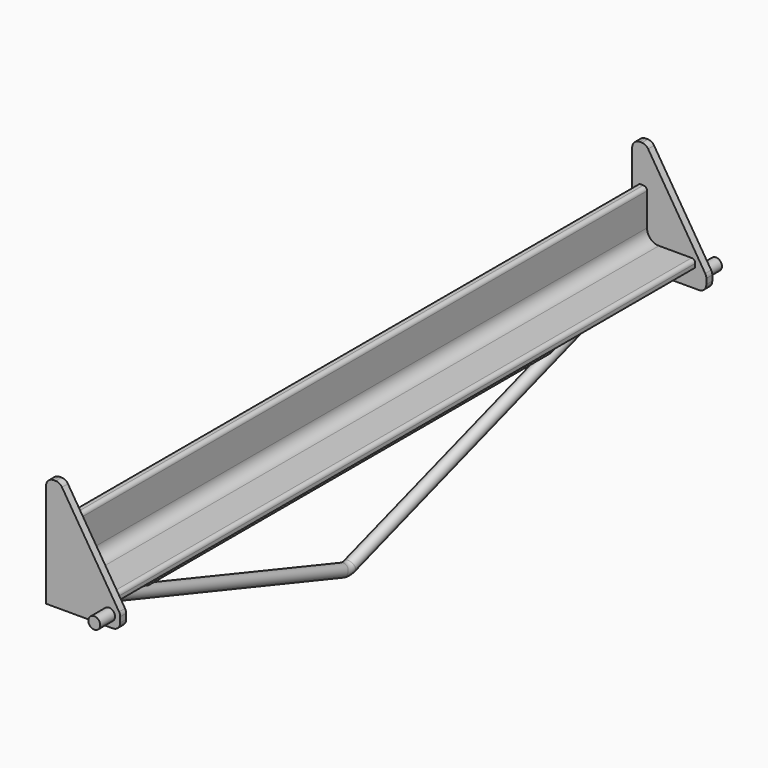
from build123d import *

# Parameters (mm, degrees)
F1_DEPTH      = 489
F1_DEPTH_BACK = 489
F2_W          = 10
F2_H          = 100
F3_DEPTH      = 489
F3_DEPTH_BACK = 489
F5_DEPTH      = 10
F6_R          = 10
F7_R          = 8
F8_DEPTH      = 25
F9_T4_DEPTH   = 788.5183031967
F9_T9_DEPTH   = 788.5183031967
F13_R         = 8


# Not quite as in the source:
# - a fillet or chamfer that OpenCascade refuses, or shapes differently, is made with other operations: its cross-section is extruded or revolved along the edge and cut away or added
# - a pattern or mirror of a feature is missing from the dataset's text; its kind, count and spacing are read off the source's solid
# - a feature names something its author has since deleted; it is built from what else it names


with BuildPart() as f1:
    # F0 (on Front) → F1 (new body, two sides)
    with BuildSketch(Plane.XZ) as f1_sk:
        with BuildLine():
            Line((5, 75), (0, 75))
            Line((0, 75), (0, 0))
            Line((0, 0), (75, 0))
            Line((75, 0), (75, 5))
            ThreePointArc((75, 5), (73.5355339059, 8.5355339059), (70, 10))
            Line((70, 10), (26, 10))
            ThreePointArc((26, 10), (14.686291501, 14.686291501), (10, 26))
            Line((10, 26), (10, 70))
            ThreePointArc((10, 70), (8.5355339059, 73.5355339059), (5, 75))
        make_face()
    extrude(amount=F1_DEPTH)
    extrude(f1_sk.sketch, amount=-F1_DEPTH_BACK)

    # F2 (on Front) → F3 (join, two sides)
    with BuildSketch(Plane.XZ) as f3_sk:
        with Locations((-5, -15)):
            Rectangle(F2_W, F2_H)
    extrude(amount=F3_DEPTH)
    extrude(f3_sk.sketch, amount=-F3_DEPTH_BACK)

    # F4 (on face) → F5 (join)
    with BuildSketch(Plane(origin=(0, 489, 0), x_dir=(-1, 0, 0), z_dir=(0, 1, 0))):
        Polygon((-90, -25), (10, -25), (10, 125), (-8.5355339059, 125), (-90, -5), align=None)
    f5 = extrude(amount=F5_DEPTH)

    # F5_copies: F5 across plane
    add(f5.mirror(Plane(origin=(0, 0, 0), x_dir=(0, 0, -1), z_dir=(0, -1, 0))))

    # F6
    f6_edges = [f1.edges().sort_by_distance(p)[0] for p in [
        (8.535534, 494, 125),
        (90, 494, -5),
        (90, 494, -25),
        (-10, 494, 125),
        (-10, -494, 125),
        (8.535534, -494, 125),
        (90, -494, -25),
        (90, -494, -5),
    ]]
    fillet(f6_edges, radius=F6_R)

    # F7 (on face) → F8 (join)
    with BuildSketch(Plane(origin=(0, 499, 0), x_dir=(-1, 0, 0), z_dir=(0, 1, 0))):
        with Locations((-75, -10)):
            Circle(F7_R)
    f8 = extrude(amount=F8_DEPTH)

    # F8_copies: F8 across plane
    add(f8.mirror(Plane(origin=(0, 0, 0), x_dir=(0, 0, -1), z_dir=(0, -1, 0))))

    # F9: chamfer of 150 x 50 on 2 edges, made by hand


with BuildPart() as f9_tool2:
    # F9_s3 → F9_t4 (new body)
    with BuildSketch(Plane.YZ.offset(-399.2591515984)):
        Polygon((-489, -15), (-339, -65), (-489, -65), align=None)
    extrude(amount=F9_T4_DEPTH)

    split(bisect_by=Plane.XY.offset(-25), keep=Keep.BOTTOM)


with BuildPart() as f1_1:
    add(f1.part)

    # F9_t1: cut F9_tool2
    add(f9_tool2.part, mode=Mode.SUBTRACT)


with BuildPart() as f9_tool7:
    # F9_s8 → F9_t9 (new body)
    with BuildSketch(Plane.YZ.offset(-399.2591515984)):
        Polygon((339, -65), (489, -15), (489, -65), align=None)
    extrude(amount=F9_T9_DEPTH)

    split(bisect_by=Plane.XY.offset(-25), keep=Keep.BOTTOM)


with BuildPart() as f1_2:
    add(f1_1.part)

    # F9_t6: cut F9_tool7
    add(f9_tool7.part, mode=Mode.SUBTRACT)

    # F14: sweep along a path in F11
    with BuildLine(Plane(origin=(-5, 0, 0), x_dir=(0, -1, 0), z_dir=(-1, 0, 0))) as f14_path:
        Line((-434.5147456835, -41.0674455892), (-6.3245553203, -183.7975090436))
        ThreePointArc((-6.3245553203, -183.7975090436), (0, -184.8238430826), (6.3245553203, -183.7975090436))
        Line((6.3245553203, -183.7975090436), (444.0904629777, -37.8755398245))
    # F13 (on line) → F14 (sweep)
    with BuildSketch(Plane(origin=(0, 378.7430374384, 126.2476791461), x_dir=(-1, 0, 0), z_dir=(0, 0.9486832981, 0.316227766))):
        with Locations((5, -176.365627053)):
            Circle(F13_R)
    sweep(path=f14_path.line)


solid = f1_2.part
